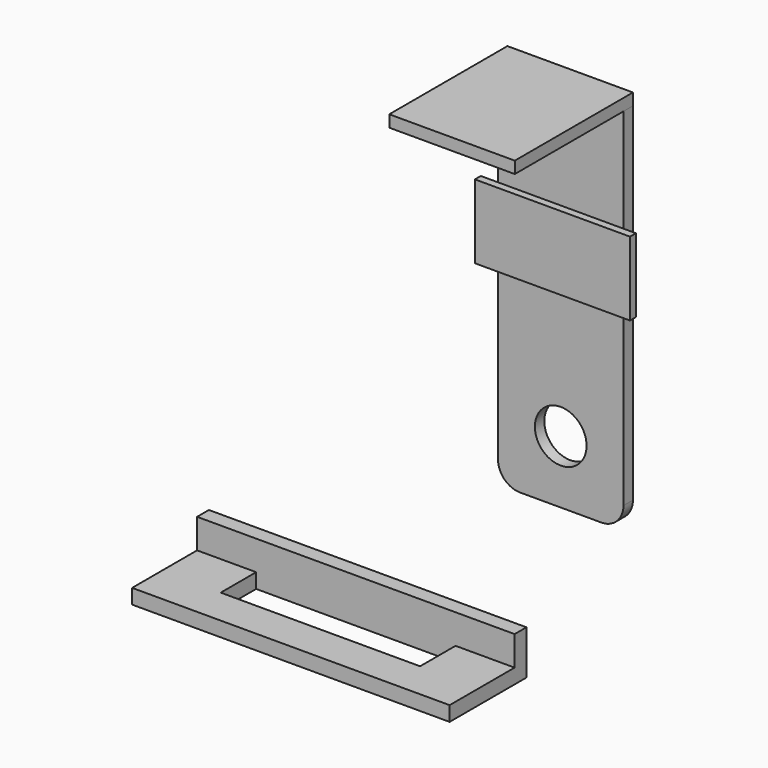
from build123d import *

# Parameters (mm, degrees)
F8_DEPTH  = 2
F7_W      = 43
F7_H      = 6
F9_DEPTH  = 2
F2_R      = 3.5
F2_W      = 17
F2_H      = 5
F2_H_2    = 28
F10_DEPTH = 1.6
F4_W      = 17
F4_H      = 20
F11_DEPTH = 1.6
F1_W      = 21
F1_H      = 10
F12_DEPTH = 1


# Not quite as in the source:
# - a feature names something its author has since deleted; it is built from what else it names


with BuildPart() as f8:
    # F5 (on Top) → F8 (new body)
    with BuildSketch(Plane.XY):
        Polygon((-5, -36.2816824913), (-13, -36.2816824913), (-13, -47.2816824913), (30, -47.2816824913), (30, -36.2816824913), (22, -36.2816824913), (22, -42.2816824913), (-5, -42.2816824913), align=None)
    extrude(amount=F8_DEPTH)

    # F7 (on line) → F9 (join)
    with BuildSketch(Plane(origin=(0, -36.2816824913, 0), x_dir=(-1, 0, 0), z_dir=(0, 1, 0))):
        with Locations((-8.5, 3)):
            Rectangle(F7_W, F7_H)
    extrude(amount=F9_DEPTH)


with BuildPart() as f10:
    # F2 (on Front) → F10 (new body)
    with BuildSketch(Plane.XZ):
        with BuildLine():
            Line((17, 17), (0, 17))
            Line((0, 17), (0, 3))
            ThreePointArc((0, 3), (0.8786796564, 0.8786796564), (3, 0))
            Line((3, 0), (14, 0))
            ThreePointArc((14, 0), (16.1213203436, 0.8786796564), (17, 3))
            Line((17, 3), (17, 17))
        make_face()
        with Locations((8.5, 8.5)):
            Circle(F2_R, mode=Mode.SUBTRACT)
        with Locations((8.5, 19.5)):
            Rectangle(F2_W, F2_H)
        with Locations((8.5, 36)):
            Rectangle(F2_W, F2_H_2)
    extrude(amount=F10_DEPTH)


with BuildPart() as f11:
    # F4 (on line) → F11 (new body)
    with BuildSketch(Plane.XY.offset(50)):
        with Locations((8.5, -10)):
            Rectangle(F4_W, F4_H)
    extrude(amount=F11_DEPTH)


with BuildPart() as f12:
    # F1 (on offset) → F12 (new body)
    with BuildSketch(Plane.XZ.offset(2)):
        with Locations((8.5, 31.2774626663)):
            Rectangle(F1_W, F1_H)
    extrude(amount=F12_DEPTH)


solid = Compound([f8.part, f10.part, f11.part, f12.part])
